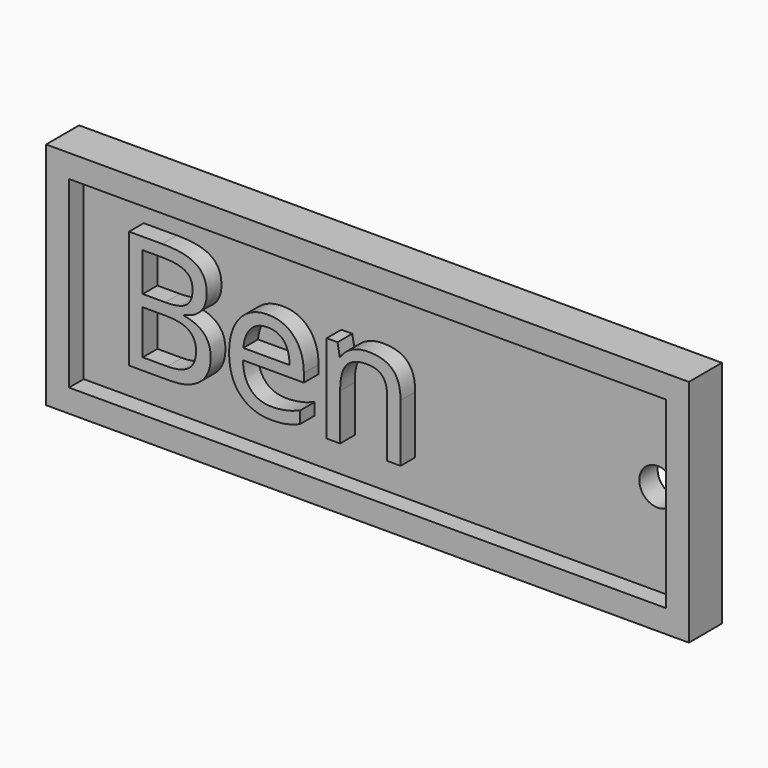
from build123d import *

# Parameters (mm, degrees)
F0_W         = 70
F0_H         = 25
F1_DEPTH     = 2.5
F2_W         = 70
F2_H         = 25
F2_W_2       = 65
F2_H_2       = 20
F3_DEPTH     = 2
F4_TEXT_SIZE = 17.9844817871
F5_DEPTH     = 2
F7_D         = 4


# Not quite as in the source:
# - Text() gives the source's letters only with a copy of the font that has no kerning and outlines rounded to 1/6400 em; it was checked with that copy


with BuildPart() as f1:
    # F0 (on Front) → F1 (new body)
    with BuildSketch(Plane.XZ):
        with Locations((35, 12.5)):
            Rectangle(F0_W, F0_H)
    extrude(amount=F1_DEPTH)

    # F2 (on face) → F3 (join)
    with BuildSketch(Plane.XZ.offset(2.5)):
        with Locations((35, 12.5)):
            Rectangle(F2_W, F2_H)
        with Locations((35, 12.5)):
            Rectangle(F2_W_2, F2_H_2, mode=Mode.SUBTRACT)
    extrude(amount=F3_DEPTH)

    # F4 (on face) → F5 (join)
    with BuildSketch(Plane.XZ.offset(2.5)):
        with Locations((7.2671994567, 6.7386748269)):
            Text('Ben', F4_TEXT_SIZE, font='Open Sans', text_align=(TextAlign.LEFT, TextAlign.BOTTOM))
    extrude(amount=F5_DEPTH)

    # F7 (through all)
    with Locations(Plane(origin=(0, 0, 0), x_dir=(-1, 0, 0), z_dir=(0, 1, 0))):
        with Locations((-65, 12.5)):
            Hole(F7_D / 2)


solid = f1.part
